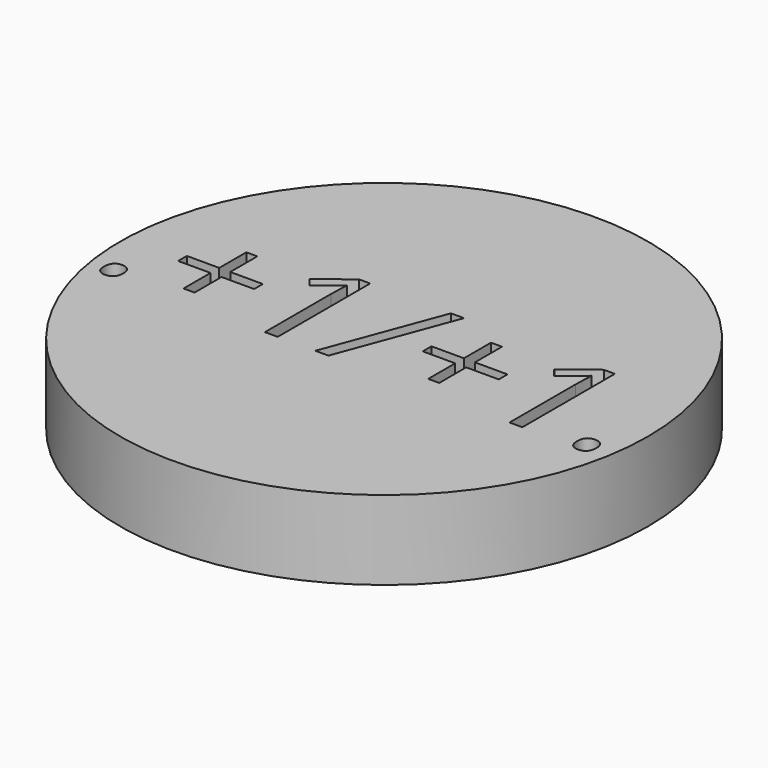
from build123d import *

# Parameters (mm, degrees)
F0_R         = 10
F1_DEPTH     = 3
F2_TEXT_SIZE = 6.1358494821
F3_DEPTH     = 2


# Not quite as in the source:
# - Text() gives the source's letters only with a copy of the font that has no kerning and outlines rounded to 1/6400 em; it was checked with that copy


with BuildPart() as f1:
    # F0 (on Top) → F1 (new body)
    with BuildSketch(Plane.XY):
        Circle(F0_R)
    extrude(amount=F1_DEPTH)

    # F2 (on face) → F3 (cut)
    with BuildSketch(Plane.XY.offset(3)):
        with Locations((-9.8255419486, -1.859764882)):
            Text('.+1/+1.', F2_TEXT_SIZE, font='Open Sans', text_align=(TextAlign.LEFT, TextAlign.BOTTOM))
    extrude(amount=-F3_DEPTH, mode=Mode.SUBTRACT)


solid = f1.part
